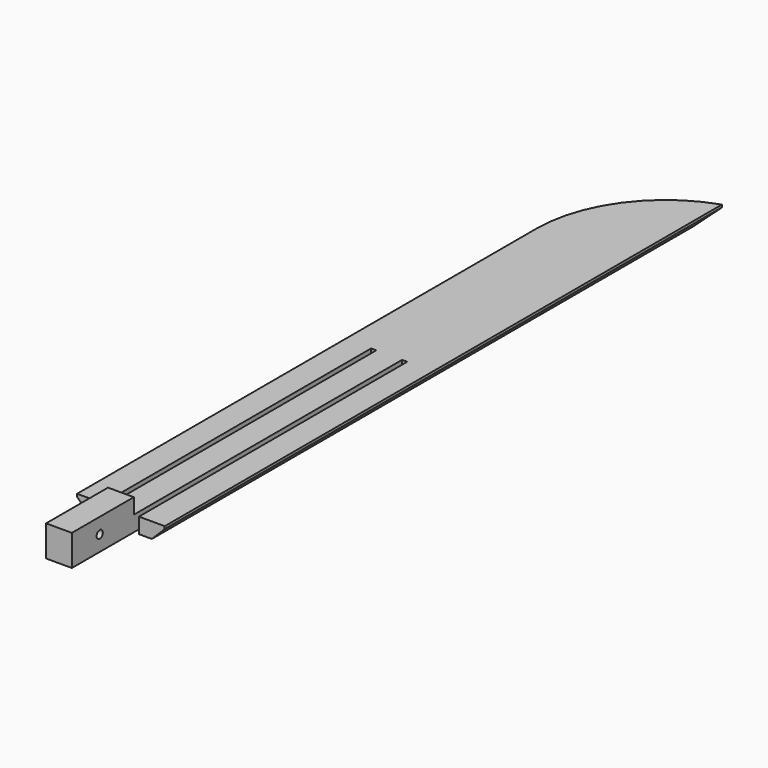
from build123d import *

# Parameters (mm, degrees)
F1_DEPTH    = 6
F2_T1_DEPTH = 242.8543856465
F3_W        = 10
F3_H        = 30
F4_DEPTH    = 6
F5_R        = 1.5
F6_DEPTH    = 10
F7_SIZE     = 5


# Not quite as in the source:
# - a fillet or chamfer that OpenCascade refuses, or shapes differently, is made with other operations: its cross-section is extruded or revolved along the edge and cut away or added


with BuildPart() as f1:
    # F0 (on Top) → F1 (new body)
    with BuildSketch(Plane.XY):
        Polygon((14.9102990106, 227.5062542017), (-19.0897009894, 227.5062542017), (-19.0897009894, -42.4937457983), (-9.0897009894, -42.4937457983), (-9.0897009894, 87.5062542017), (-7.0897009894, 87.5062542017), (-7.0897009894, -72.4937457983), (2.9102990106, -72.4937457983), (2.9102990106, 87.5062542017), (4.9102990106, 87.5062542017), (4.9102990106, -42.4937457983), (14.9102990106, -42.4937457983), align=None)
    extrude(amount=F1_DEPTH)

    # F2: fillet of radius 50 on 1 edges, made by hand

    # F2_s2 → F2_t1 (cut)
    with BuildSketch(Plane.XY.offset(-118.4271928233)):
        with BuildLine():
            ThreePointArc((14.9102990106, 227.5062542017), (-9.7098930126, 209.2901365467), (-19.0897009894, 180.1353770724))
            Line((-19.0897009894, 180.1353770724), (-19.0897009894, 227.5062542017))
            Line((-19.0897009894, 227.5062542017), (14.9102990106, 227.5062542017))
        make_face()
    extrude(amount=F2_T1_DEPTH, mode=Mode.SUBTRACT)

    # F3 (on face) → F4 (join)
    with BuildSketch(Plane.XY.offset(6)):
        with Locations((-2.0897009894, -57.4937457983)):
            Rectangle(F3_W, F3_H)
    extrude(amount=F4_DEPTH)

    # F5 (on face) → F6 (cut, through all)
    with BuildSketch(Plane(origin=(-7.0897009894, 0, 0), x_dir=(0, -1, 0), z_dir=(-1, 0, 0))):
        with Locations((59.0019002557, 6)):
            Circle(F5_R)
    extrude(amount=-F6_DEPTH, mode=Mode.SUBTRACT)

    # F7
    f7_edges = [f1.edges().sort_by_distance(p)[0] for p in [
        (14.910299, 92.506254, 0),
        (-19.089701, 68.820816, 0),
        (-9.709893, 209.290137, 0),
    ]]
    chamfer(f7_edges, length=F7_SIZE)


solid = f1.part
